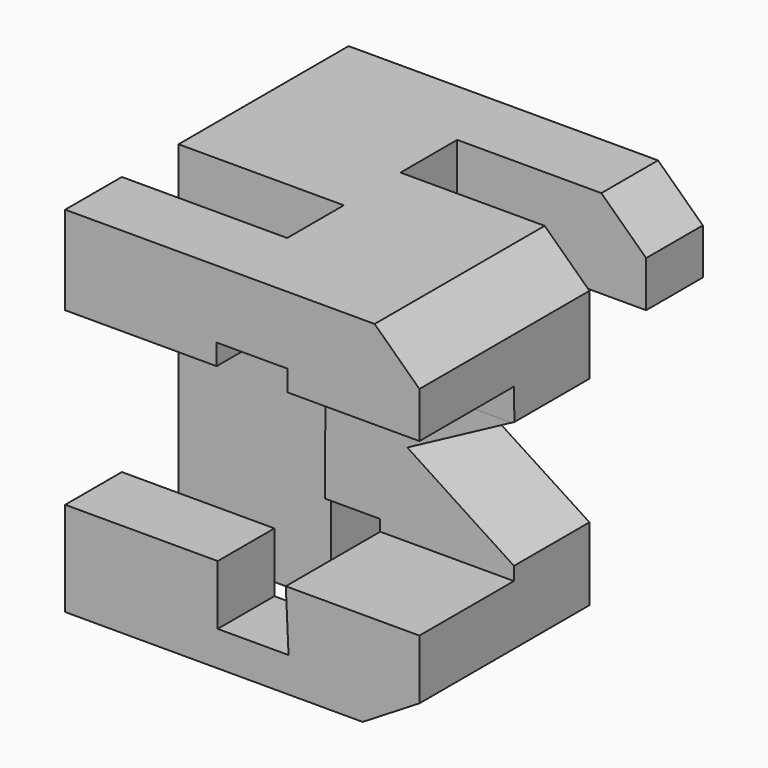
from build123d import *

# Parameters (mm, degrees)
F0_W      = 38.1
F0_H      = 38.1
F1_DEPTH  = 38.1
F5_W      = 12.7
F5_H      = 28.575
F6_DEPTH  = 38.1
F7_W      = 20.32
F7_H      = 7.62
F7_W_2    = 17.78
F8_DEPTH  = 38.1
F9_W      = 7.62
F9_H      = 7.62
F10_DEPTH = 76.2


with BuildPart() as f1:
    # F0 (on Front) → F1 (new body)
    with BuildSketch(Plane.XZ):
        with Locations((19.05, 19.05)):
            Rectangle(F0_W, F0_H)
    extrude(amount=F1_DEPTH)

    # F5 (on offset) → F6 (cut)
    with BuildSketch(Plane.YZ.offset(38.1)):
        with Locations((-6.35, 14.2875)):
            Rectangle(F5_W, F5_H)
        Polygon((-25.4, 28.575), (-38.1, 28.575), (-38.1, 10.16), (-25.4, 10.16), (-25.324332, 25.021608), align=None)
    extrude(amount=-F6_DEPTH, mode=Mode.SUBTRACT)

    # F7 (on offset) → F8 (cut)
    with BuildSketch(Plane.XY.offset(38.1)):
        with Locations((27.94, -11.43)):
            Rectangle(F7_W, F7_H)
        with Locations((8.89, -26.67)):
            Rectangle(F7_W_2, F7_H)
    extrude(amount=-F8_DEPTH, mode=Mode.SUBTRACT)

    # F9 (on offset) → F10 (cut)
    with BuildSketch(Plane.XZ.offset(76.2)):
        with Locations((20.097828, 27.007606)):
            Rectangle(F9_W, F9_H)
        Polygon((38.1, 38.1), (33.282343, 38.1), (38.1, 33.511519), align=None)
        Polygon((38.1, 11.594454), (38.1, 25.190067), (26.601743, 19.05), align=None)
        Polygon((38.1, 3.741816), (31.993106, 0), (38.1, 0), align=None)
        Polygon((23.671653, 11.360046), (16.403263, 11.360046), (16.403263, 3.740046), (24.023263, 3.740046), align=None)
    extrude(amount=-F10_DEPTH, mode=Mode.SUBTRACT)


solid = f1.part
